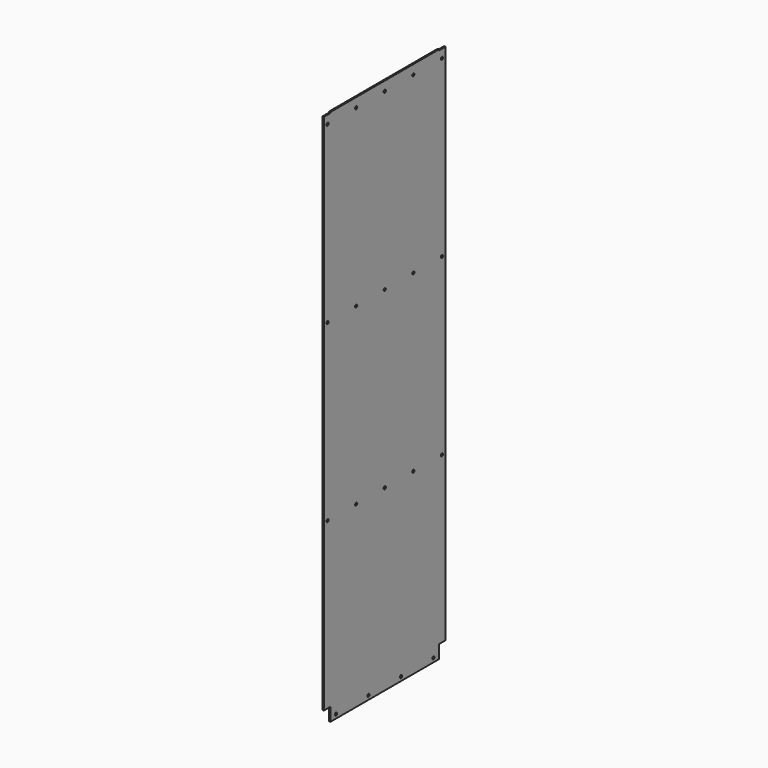
from build123d import *

# Parameters (mm, degrees)
F0_W     = 311.15
F0_H     = 1097.3562
F1_DEPTH = 1.51892
F2_W     = 16.51
F2_H     = 27.1526
F3_DEPTH = 3.03784
F4_W     = 16.51
F4_H     = 1.905
F5_DEPTH = 3.03784
F7_D     = 5.6134


# Not quite as in the source:
# - a pattern or mirror of a feature is missing from the dataset's text; its kind, count and spacing are read off the source's solid
# - a feature names something its author has since deleted; it is built from what else it names


with BuildPart() as f1:
    # F0 (on Right) → F1 (new body, symmetric)
    with BuildSketch(Plane.YZ):
        Rectangle(F0_W, F0_H)
    extrude(amount=F1_DEPTH, both=True)

    # F2 (on face) → F3 (cut, through all)
    with BuildSketch(Plane.YZ.offset(1.51892)):
        with Locations((-147.32, -535.1018)):
            Rectangle(F2_W, F2_H)
    f3 = extrude(amount=-F3_DEPTH, mode=Mode.SUBTRACT)

    # F3_copies: F3 across plane
    add(f3.mirror(Plane.ZX), mode=Mode.SUBTRACT)

    # F4 (on face) → F5 (cut, through all)
    with BuildSketch(Plane.YZ.offset(1.51892)):
        with Locations((-147.32, 547.7256)):
            Rectangle(F4_W, F4_H)
        with Locations((147.32, 547.7256)):
            Rectangle(F4_W, F4_H)
    extrude(amount=-F5_DEPTH, mode=Mode.SUBTRACT)

    # F7 (through all)
    with Locations(Plane(origin=(-1.51892, 0, 0), x_dir=(0, -1, 0), z_dir=(-1, 0, 0))):
        with Locations((124.587, -540.5501), (41.529, -540.5501), (-41.529, -540.5501), (-124.587, -540.5501), (146.05, -183.8071), (146.05, 172.9359), (73.025, 172.9359), (0, 172.9359), (-73.025, 172.9359), (-146.05, 172.9359), (-146.05, -183.8071), (-73.025, -183.8071), (0, -183.8071), (73.025, -183.8071), (146.05, 529.6789), (73.025, 529.6789), (0, 529.6789), (-73.025, 529.6789), (-146.05, 529.6789)):
            Hole(F7_D / 2)


solid = f1.part
